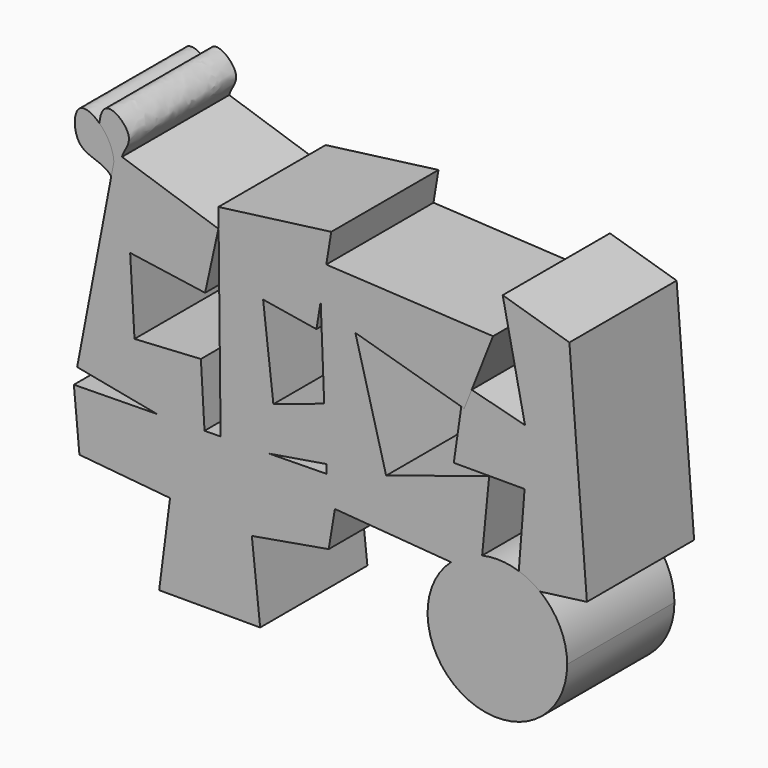
from build123d import *

# Parameters (mm, degrees)
F1_DEPTH = 25
F2_DEPTH = 25


# Not quite as in the source:
# - a feature names something its author has since deleted; it is built from what else it names


with BuildPart() as f1:
    # F0 (on Front) → F1 (new body)
    with BuildSketch(Plane.XZ):
        Polygon((-47.5800185116, 25.1394304663), (-48.7721934915, 25.5340393633), (-49.0936644847, 23.8471837339), (-49.580643877, 21.2918554258), (-55.9416088431, -12.0860535841), (-41.040990114, -14.9524709667), (-32.1869384028, -14.8245029716), (-32.865631272, -3.2554731287), (-45.2441488891, -3.9816542997), (-46.057574451, 9.8840352148), (-32.0782847703, 7.8648040071), (-29.5930765569, 19.1857680893), align=None)
        Polygon((-29.5930765569, 22.7760467678), (-29.1833552576, -14.7810920536), (-20.1023506464, -14.6498438984), (-9.4787493108, -12.890154367), (-9.8642086396, -3.1116086064), (-19.3415973336, -6.2698121183), (-21.2589813071, 10.2837849514), (-11.3086648334, 8.6555517214), (-10.5184212473, 13.4848191924), (-10.7724191621, 19.9283789843), (-9.4753039798, 19.8594261832), (-8.5467311277, 25.5340393633), align=None)
        Polygon((16.2491034716, 4.5750387944), (17.646368447, 8.115980815), (16.2491034716, 8.4770983085), (15.7077395213, 4.7308423127), align=None)
        Polygon((-32.0782847703, -16.6766177863), (-41.040990114, -14.9524709667), (-56.5548166633, -15.1766929775), (-55.5187724531, -26.3442061841), (-38.6174283922, -27.9604550451), (-40.6492874026, -43.7535122037), (-21.8084454536, -43.7535122037), (-23.3626682311, -29.2172543705), (-9.0179853141, -26.7231296748), (-7.8705830286, -19.7518104097), (-9.2123951763, -19.6471735835), (-9.415472877, -14.4953859884), (-20.1023506464, -14.6498438984), (-29.1684046388, -16.151541844), (-29.1833552576, -14.7810920536), (-32.1869384028, -14.8245029716), align=None)
        Polygon((-32.1869384028, -14.8245029716), (-41.040990114, -14.9524709667), (-32.0782847703, -16.6766177863), align=None)
        Polygon((-6.999686826, -14.4604705274), (-9.415472877, -14.4953859884), (-9.2123951763, -19.6471735835), (-7.8705830286, -19.7518104097), align=None)
        Polygon((-9.8642086396, -3.1116086064), (-9.4787493108, -12.890154367), (-9.0938955545, -12.8264073282), (-8.4957480431, -2.6555887889), align=None)
        Polygon((-20.1023506464, -14.6498438984), (-29.1833552576, -14.7810920536), (-29.1684046388, -16.151541844), align=None)
        with BuildLine():
            Line((19.2611534148, -21.8675900251), (13.7905507625, -21.4409829924))
            ThreePointArc((13.7905507625, -21.4409829924), (17.104977269, -43.0510244401), (35.4600015258, -31.1736341978))
            ThreePointArc((35.4600015258, -31.1736341978), (34.1260357026, -25.4327233148), (30.3974732406, -20.8681483563))
            Line((30.3974732406, -20.8681483563), (26.2241458364, -21.4150369417))
            Line((26.2241458364, -21.4150369417), (26.4307223653, -18.7800200512))
            ThreePointArc((26.4307223653, -18.7800200512), (23.0326147125, -18.1667508172), (19.5928003292, -18.4682666253))
            Line((19.5928003292, -18.4682666253), (19.2611534148, -21.8675900251))
        make_face()
        with BuildLine():
            ThreePointArc((19.5928003292, -18.4682666253), (16.5026063559, -19.5855930916), (13.7905507625, -21.4409829924))
            Line((13.7905507625, -21.4409829924), (19.2611534148, -21.8675900251))
            Line((19.2611534148, -21.8675900251), (19.5928003292, -18.4682666253))
        make_face()
        with BuildLine():
            ThreePointArc((30.3974732406, -20.8681483563), (28.504638765, -19.6520864201), (26.4307223653, -18.7800200512))
            Line((26.4307223653, -18.7800200512), (26.2241458364, -21.4150369417))
            Line((26.2241458364, -21.4150369417), (30.3974732406, -20.8681483563))
        make_face()
        Polygon((-10.5184212473, 13.4848191924), (-9.4753039798, 19.8594261832), (-10.7724191621, 19.9283789843), align=None)
        with BuildLine():
            Line((-9.0938955545, -12.8264073282), (-9.4787493108, -12.890154367))
            Line((-9.4787493108, -12.890154367), (-9.415472877, -14.4953859884))
            Line((-9.415472877, -14.4953859884), (-6.999686826, -14.4604705274))
            Line((-6.999686826, -14.4604705274), (-7.8705830286, -19.7518104097))
            Line((-7.8705830286, -19.7518104097), (13.7905507625, -21.4409829924))
            ThreePointArc((13.7905507625, -21.4409829924), (16.5026063559, -19.5855930916), (19.5928003292, -18.4682666253))
            Line((19.5928003292, -18.4682666253), (20.9103631787, -4.9634757452))
            Line((20.9103631787, -4.9634757452), (1.6931692371, -11.1684147269))
            Line((1.6931692371, -11.1684147269), (-4.0499549359, 10.4170693085))
            Line((-4.0499549359, 10.4170693085), (15.7077395213, 4.7308423127))
            Line((15.7077395213, 4.7308423127), (16.2491034716, 8.4770983085))
            Line((16.2491034716, 8.4770983085), (17.646368447, 8.115980815))
            Line((17.646368447, 8.115980815), (21.6279253364, 18.2060226798))
            Line((21.6279253364, 18.2060226798), (-9.4753039798, 19.8594261832))
            Line((-9.4753039798, 19.8594261832), (-10.5184212473, 13.4848191924))
            Line((-10.5184212473, 13.4848191924), (-9.8642086396, -3.1116086064))
            Line((-9.8642086396, -3.1116086064), (-8.4957480431, -2.6555887889))
            Line((-8.4957480431, -2.6555887889), (-9.0938955545, -12.8264073282))
        make_face()
        with BuildLine():
            Line((-49.0936644847, 23.8471837339), (-48.7721934915, 25.5340393633))
            Line((-48.7721934915, 25.5340393633), (-47.5800185116, 25.1394304663))
            add(Edge.make_bspline(
                [(-51.7847523134, 29.3005192438), (-51.6938141857, 30.6509644727), (-50.5313148062, 33.9628150244), (-44.6471394652, 28.923709997), (-47.2538191761, 26.3599821773), (-47.5800185116, 25.1394304663)],
                knots=[0.3213691305, 0.3213691305, 0.3213691305, 0.3213691305, 0.4879946472, 0.7538353497, 0.9672352852, 0.9672352852, 0.9672352852, 0.9672352852], degree=3))
            add(Edge.make_bspline(
                [(-51.7847523091, 29.300519245), (-50.5127452087, 28.0918020949), (-49.3916383719, 26.2759976867), (-49.1380687641, 24.327482226)],
                knots=[0.8017018355, 0.8017018355, 0.8017018355, 0.8017018355, 0.9850135384, 0.9850135384, 0.9850135384, 0.9850135384], degree=3))
            add(Edge.make_bspline(
                [(-49.1380687641, 24.327482226), (-49.117338439, 24.1681833284), (-49.1024064842, 24.0079974281), (-49.0936644847, 23.8471837339)],
                knots=[0.9850135384, 0.9850135384, 0.9850135384, 0.9850135384, 1, 1, 1, 1], degree=3))
        make_face()
    extrude(amount=-F1_DEPTH)


with BuildPart() as f2:
    # F0 (on Front) → F2 (new body)
    with BuildSketch(Plane.XZ):
        with BuildLine():
            Line((27.5915823877, 5.5456804112), (17.646368447, 8.115980815))
            Line((17.646368447, 8.115980815), (16.2491034716, 4.5750387944))
            Line((16.2491034716, 4.5750387944), (15.7077395213, 4.7308423127))
            Line((15.7077395213, 4.7308423127), (14.3068330362, -4.9634757452))
            Line((14.3068330362, -4.9634757452), (20.9103631787, -4.9634757452))
            Line((20.9103631787, -4.9634757452), (27.5138933212, -4.9634757452))
            Line((27.5138933212, -4.9634757452), (26.4307223653, -18.7800200512))
            ThreePointArc((26.4307223653, -18.7800200512), (28.504638765, -19.6520864201), (30.3974732406, -20.8681483563))
            Line((30.3974732406, -20.8681483563), (39.138417691, -19.7227019817))
            Line((39.138417691, -19.7227019817), (35.8731001616, 21.8121092767))
            Line((35.8731001616, 21.8121092767), (23.4314221889, 25.5340393633))
            Line((23.4314221889, 25.5340393633), (27.5915823877, 5.5456804112))
        make_face()
    extrude(amount=-F2_DEPTH)


with BuildPart() as f2b:
    # F0 (on Front) → F2, piece 2 (new body)
    with BuildSketch(Plane.XZ):
        with BuildLine():
            Line((-49.580643877, 21.2918554258), (-49.0936644847, 23.8471837339))
            add(Edge.make_bspline(
                [(-49.1380687641, 24.327482226), (-49.117338439, 24.1681833284), (-49.1024064842, 24.0079974281), (-49.0936644847, 23.8471837339)],
                knots=[0.9850135384, 0.9850135384, 0.9850135384, 0.9850135384, 1, 1, 1, 1], degree=3))
            add(Edge.make_bspline(
                [(-49.1380687641, 24.327482226), (-50.1405346839, 24.9125897933), (-51.5910596929, 25.7731299005), (-51.8409229757, 28.4663762406), (-51.7847523134, 29.3005192438)],
                knots=[0, 0, 0, 0, 0.218447882, 0.3213691305, 0.3213691305, 0.3213691305, 0.3213691305], degree=3))
            add(Edge.make_bspline(
                [(-49.580643877, 21.2918554258), (-51.170963794, 23.2717152685), (-56.7265800947, 22.6369556897), (-56.7181417239, 32.0928453298), (-53.0149801468, 30.4695359001), (-51.7847523091, 29.300519245)],
                knots=[0, 0, 0, 0, 0.3229597325, 0.6244110329, 0.8017018355, 0.8017018355, 0.8017018355, 0.8017018355], degree=3))
        make_face()
        with BuildLine():
            add(Edge.make_bspline(
                [(-51.7847523091, 29.300519245), (-50.5127452087, 28.0918020949), (-49.3916383719, 26.2759976867), (-49.1380687641, 24.327482226)],
                knots=[0.8017018355, 0.8017018355, 0.8017018355, 0.8017018355, 0.9850135384, 0.9850135384, 0.9850135384, 0.9850135384], degree=3))
            add(Edge.make_bspline(
                [(-49.1380687641, 24.327482226), (-50.1405346839, 24.9125897933), (-51.5910596929, 25.7731299005), (-51.8409229757, 28.4663762406), (-51.7847523134, 29.3005192438)],
                knots=[0, 0, 0, 0, 0.218447882, 0.3213691305, 0.3213691305, 0.3213691305, 0.3213691305], degree=3))
        make_face()
    extrude(amount=-F2_DEPTH)


solid = Compound([f1.part, f2.part, f2b.part])
